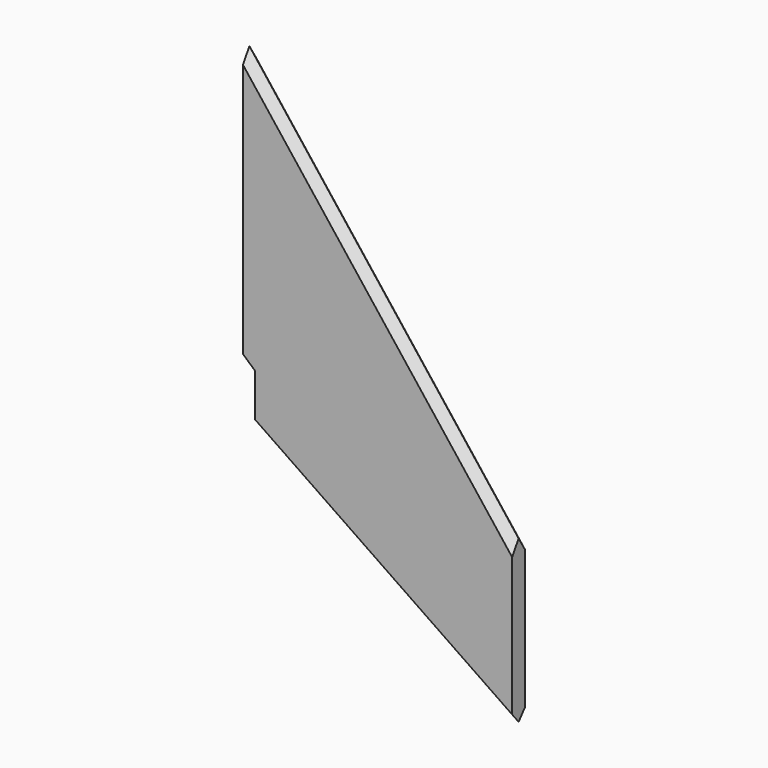
from build123d import *

# Parameters (mm, degrees)
F1_DEPTH = 3
F2_SIZE  = 1.49999
F4_DEPTH = 4


# Not quite as in the source:
# - a fillet or chamfer is up to 0.001 mm smaller than in the source, because OpenCascade refuses the exact size


with BuildPart() as f1:
    # F0 (on Front) → F1 (new body)
    with BuildSketch(Plane.XZ):
        Polygon((0, 60), (0, 0), (50, -34.25), (50, -4.25), align=None)
    extrude(amount=F1_DEPTH)

    # F2 (size 1.5 in the source; OpenCascade refuses exactly that, so slightly less here)
    f2_edges = [f1.edges().sort_by_distance(p)[0] for p in [
        (25, -3, 27.875),
        (25, 0, 27.875),
        (25, -3, -17.125),
        (25, 0, -17.125),
    ]]
    chamfer(f2_edges, length=F2_SIZE)

    # F3 (on Front) → F4 (cut, symmetric)
    with BuildSketch(Plane.XZ):
        Polygon((2.25, 8.25), (0, 10.25), (0, -5), (2.25, -5), align=None)
    extrude(amount=F4_DEPTH, both=True, mode=Mode.SUBTRACT)


solid = f1.part
